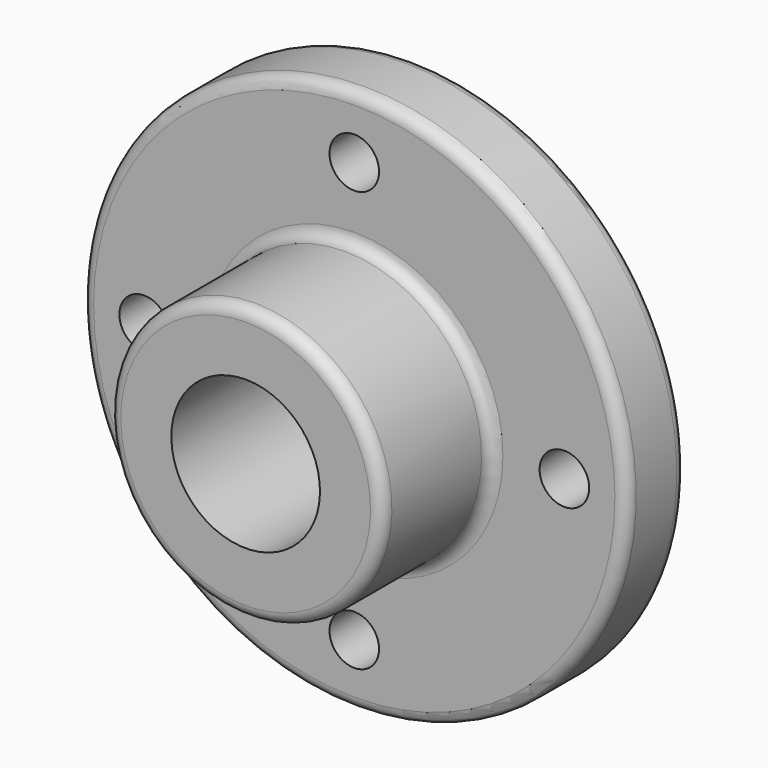
from build123d import *

# Parameters (mm, degrees)
F2_R            = 3.048
F3_R            = 6.35
F4_DEPTH        = 19.051
F4_COPIES_COUNT = 4


# Not quite as in the source:
# - a pattern or mirror of a feature is missing from the dataset's text; its kind, count and spacing are read off the source's solid


with BuildPart() as f1:
    # F0 (on Right) → F1 (revolve)
    with BuildSketch(Plane.YZ):
        Polygon((-53.848, 19.05), (0, 19.05), (0, 69.85), (-19.05, 69.85), (-19.05, 35.052), (-53.848, 35.052), align=None)
    revolve(axis=Axis((0, -30.1634762436, 0), (0, -1, 0)))

    # F2
    f2_edges = [f1.edges().sort_by_distance(p)[0] for p in [
        (0, -53.848, -35.052),
        (0, -19.05, -35.052),
        (0, -19.05, -69.85),
        (0, 0, -69.85),
    ]]
    fillet(f2_edges, radius=F2_R)

    # F3 (on face) → F4 (cut, through all)
    with BuildSketch(Plane.XZ.offset(19.05)):
        with Locations((0, 53.848)):
            Circle(F3_R)
    f4 = extrude(amount=-F4_DEPTH, mode=Mode.SUBTRACT)

    # F4_copies: F4 ×4 about axis
    f4_copies_axis = Axis((0, 0, 0), (0, 1, 0))
    for i in range(1, F4_COPIES_COUNT):
        add(f4.rotate(f4_copies_axis, i * 360 / F4_COPIES_COUNT), mode=Mode.SUBTRACT)


solid = f1.part
